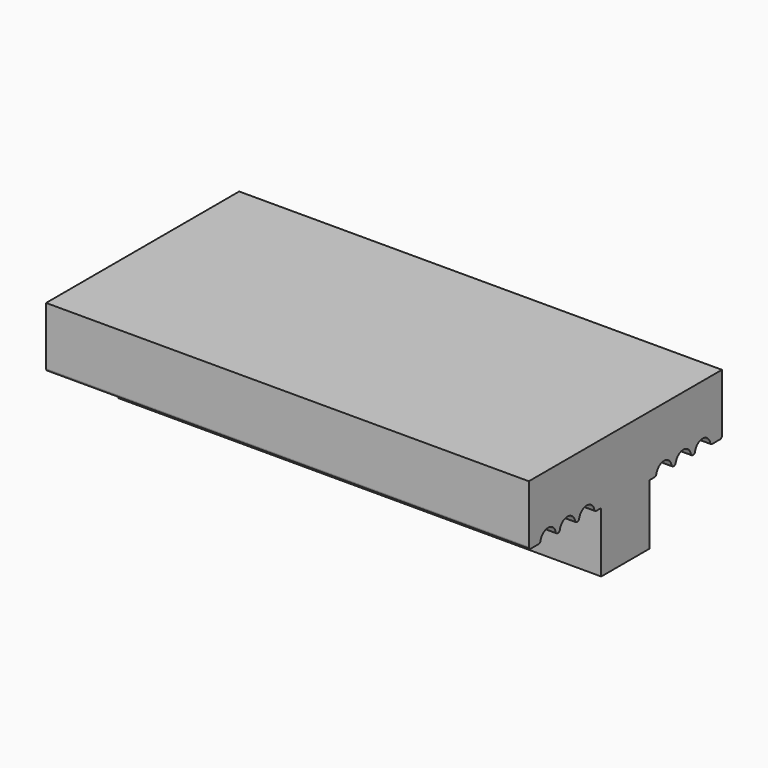
from build123d import *

# Parameters (mm, degrees)
F1_DEPTH = 50.8
F2_R     = 0.254


with BuildPart() as f1:
    # F0 (on Right) → F1 (new body)
    with BuildSketch(Plane.YZ):
        with BuildLine():
            Line((0, 6.35), (0, 0))
            Line((0, 0), (1.524, 0))
            ThreePointArc((1.524, 0), (2.54, 1.016), (3.556, 0))
            Line((3.556, 0), (4.064, 0))
            ThreePointArc((4.064, 0), (5.08, 1.016), (6.096, 0))
            Line((6.096, 0), (6.604, 0))
            ThreePointArc((6.604, 0), (7.62, 1.016), (8.636, 0))
            Line((8.636, 0), (9.525, 0))
            Line((9.525, 0), (9.525, -6.35))
            Line((9.525, -6.35), (15.875, -6.35))
            Line((15.875, -6.35), (15.875, 0))
            Line((15.875, 0), (16.764, 0))
            ThreePointArc((16.764, 0), (17.78, 1.016), (18.796, 0))
            Line((18.796, 0), (19.304, 0))
            ThreePointArc((19.304, 0), (20.32, 1.016), (21.336, 0))
            Line((21.336, 0), (21.844, 0))
            ThreePointArc((21.844, 0), (22.86, 1.016), (23.876, 0))
            Line((23.876, 0), (25.4, 0))
            Line((25.4, 0), (25.4, 6.35))
            Line((25.4, 6.35), (0, 6.35))
        make_face()
    extrude(amount=F1_DEPTH)

    # F2
    f2_edges = [f1.edges().sort_by_distance(p)[0] for p in [
        (25.4, 23.876, 0),
        (25.4, 25.4, 0),
        (25.4, 21.336, 0),
        (25.4, 18.796, 0),
        (25.4, 6.604, 0),
        (25.4, 4.064, 0),
        (25.4, 1.524, 0),
        (25.4, 0, 0),
        (25.4, 3.556, 0),
        (25.4, 6.096, 0),
        (25.4, 8.636, 0),
        (25.4, 16.764, 0),
        (25.4, 19.304, 0),
        (25.4, 21.844, 0),
    ]]
    fillet(f2_edges, radius=F2_R)


solid = f1.part
